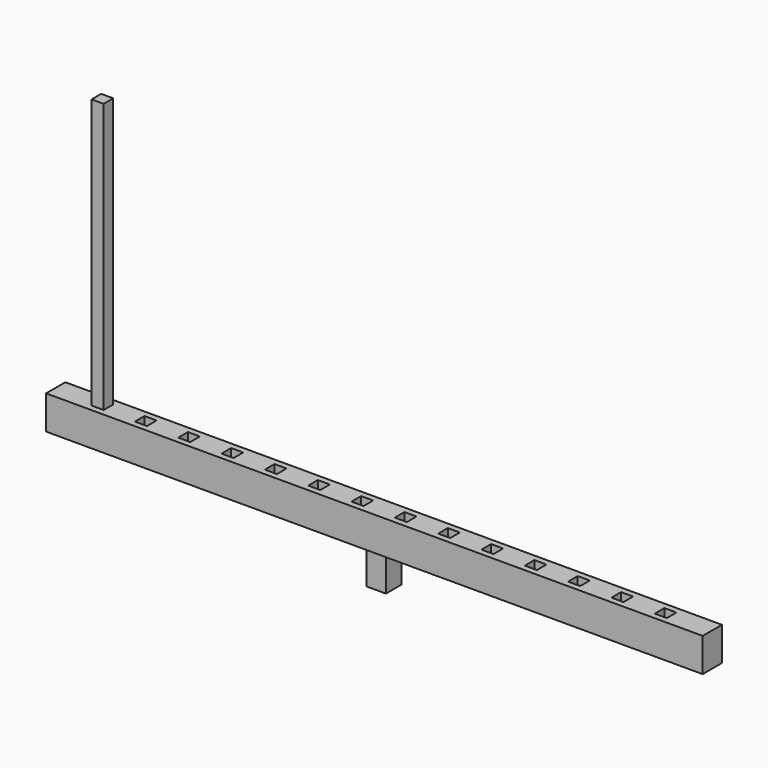
from build123d import *

# Parameters (mm, degrees)
F0_W     = 1732.3054
F0_H     = 63.5
F0_W_2   = 31.75
F0_H_2   = 31.75
F1_DEPTH = 88.9
F3_W     = 50.8
F3_H     = 50.8
F4_DEPTH = 88.9
F2_W     = 31.75
F2_H     = 31.75
F5_DEPTH = 711.2


with BuildPart() as f1:
    # F0 (on Top) → F1 (new body)
    with BuildSketch(Plane.XY):
        Rectangle(F0_W, F0_H)
        with Locations((-742.95, 0)):
            Rectangle(F0_W_2, F0_H_2, mode=Mode.SUBTRACT)
        with Locations((-628.65, 0)):
            Rectangle(F0_W_2, F0_H_2, mode=Mode.SUBTRACT)
        with Locations((-514.35, 0)):
            Rectangle(F0_W_2, F0_H_2, mode=Mode.SUBTRACT)
        with Locations((-400.05, 0)):
            Rectangle(F0_W_2, F0_H_2, mode=Mode.SUBTRACT)
        with Locations((-285.75, 0)):
            Rectangle(F0_W_2, F0_H_2, mode=Mode.SUBTRACT)
        with Locations((-171.45, 0)):
            Rectangle(F0_W_2, F0_H_2, mode=Mode.SUBTRACT)
        with Locations((-57.15, 0)):
            Rectangle(F0_W_2, F0_H_2, mode=Mode.SUBTRACT)
        with Locations((57.15, 0)):
            Rectangle(F0_W_2, F0_H_2, mode=Mode.SUBTRACT)
        with Locations((171.45, 0)):
            Rectangle(F0_W_2, F0_H_2, mode=Mode.SUBTRACT)
        with Locations((285.75, 0)):
            Rectangle(F0_W_2, F0_H_2, mode=Mode.SUBTRACT)
        with Locations((400.05, 0)):
            Rectangle(F0_W_2, F0_H_2, mode=Mode.SUBTRACT)
        with Locations((514.35, 0)):
            Rectangle(F0_W_2, F0_H_2, mode=Mode.SUBTRACT)
        with Locations((628.65, 0)):
            Rectangle(F0_W_2, F0_H_2, mode=Mode.SUBTRACT)
        with Locations((742.95, 0)):
            Rectangle(F0_W_2, F0_H_2, mode=Mode.SUBTRACT)
    extrude(amount=F1_DEPTH)

    # F3 (on face) → F4 (join)
    with BuildSketch(Plane(origin=(0, 0, 0), x_dir=(1, 0, 0), z_dir=(0, 0, -1))):
        Rectangle(F3_W, F3_H)
    extrude(amount=F4_DEPTH)


with BuildPart() as f5:
    # F2 (on face) → F5 (new body)
    with BuildSketch(Plane.XY.offset(88.9)):
        with Locations((-742.95, 0)):
            Rectangle(F2_W, F2_H)
    extrude(amount=F5_DEPTH)


solid = Compound([f1.part, f5.part])
